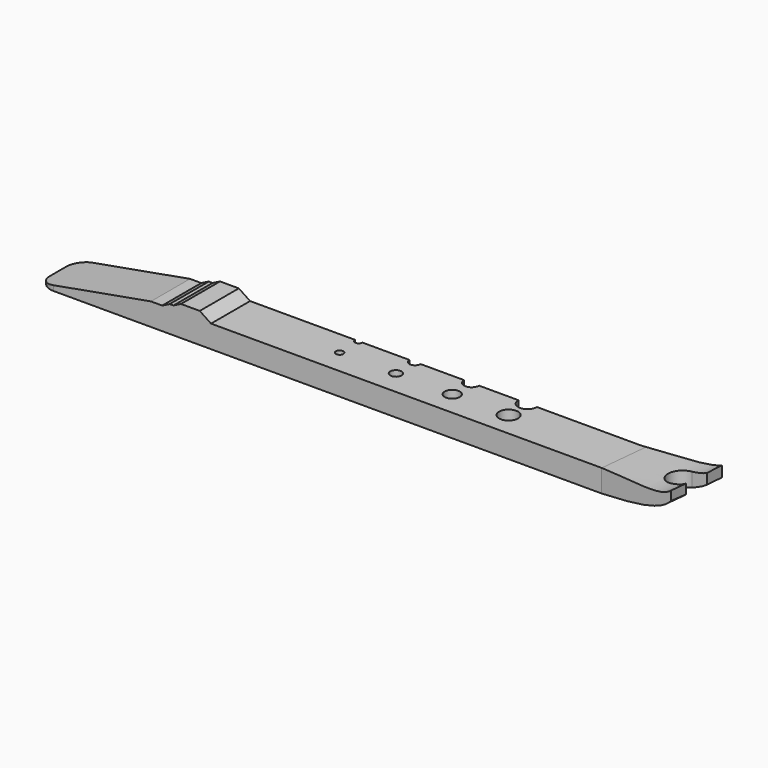
from build123d import *

# Parameters (mm, degrees)
F0_R     = 1
F0_R_2   = 1.5
F0_R_3   = 2
F1_DEPTH = 6
F3_DEPTH = 8
F5_DEPTH = 25
F7_DEPTH = 25
F9_DEPTH = 13


# Not quite as in the source:
# - a feature names something its author has since deleted; it is built from what else it names


with BuildPart() as f1:
    # F0 (on Top) → F1 (new body)
    with BuildSketch(Plane.XY):
        with BuildLine():
            Line((-42.1966487169, -12.8954221606), (-42.1966487169, -25.8954221606))
            Line((-42.1966487169, -25.8954221606), (17.9292613268, -25.8954221606))
            Line((17.9292613268, -25.8954221606), (47.9292613268, -25.8954221606))
            Line((47.9292613268, -25.8954221606), (47.9292613268, -12.8954221606))
            Line((47.9292613268, -12.8954221606), (20.3033512831, -12.8954221606))
            ThreePointArc((20.3033512831, -12.8954221606), (17.8033512831, -15.3954221606), (15.3033512831, -12.8954221606))
            Line((15.3033512831, -12.8954221606), (4.8663063049, -12.8954221606))
            ThreePointArc((4.8663063049, -12.8954221606), (2.8663063049, -14.8954221606), (0.8663063049, -12.8954221606))
            Line((0.8663063049, -12.8954221606), (-10.6966487169, -12.8954221606))
            ThreePointArc((-10.6966487169, -12.8954221606), (-12.1966487169, -14.3954221606), (-13.6966487169, -12.8954221606))
            Line((-13.6966487169, -12.8954221606), (-26.1966487169, -12.8954221606))
            ThreePointArc((-26.1966487169, -12.8954221606), (-27.1966487169, -13.8954221606), (-28.1966487169, -12.8954221606))
            Line((-28.1966487169, -12.8954221606), (-42.1966487169, -12.8954221606))
        make_face()
        with Locations((-27.0707386732, -19.3954221606)):
            Circle(F0_R, mode=Mode.SUBTRACT)
        with Locations((-12.0707386732, -19.3954221606)):
            Circle(F0_R_2, mode=Mode.SUBTRACT)
        with Locations((2.9292613268, -19.3954221606)):
            Circle(F0_R_3, mode=Mode.SUBTRACT)
        with BuildLine():
            ThreePointArc((20.4292613268, -19.3954221606), (19.6970282798, -21.1631891136), (17.9292613268, -21.8954221606))
            ThreePointArc((17.9292613268, -21.8954221606), (16.1614943738, -17.6276552077), (20.4292613268, -19.3954221606))
        make_face(mode=Mode.SUBTRACT)
        with BuildLine():
            ThreePointArc((-102.1092408178, -21.9157785711), (-100.9305134828, -24.7310372299), (-98.109292616, -25.8954221606))
            Line((-98.109292616, -25.8954221606), (-42.1966487169, -25.8954221606))
            Line((-42.1966487169, -25.8954221606), (-42.1966487169, -12.8954221606))
            Line((-42.1966487169, -12.8954221606), (-98.1347384587, -12.8954221606))
            ThreePointArc((-98.1347384587, -12.8954221606), (-100.9703535279, -14.0742012939), (-102.1346866604, -16.9157785711))
            Line((-102.1346866604, -16.9157785711), (-102.1092408178, -21.9157785711))
        make_face()
    extrude(amount=F1_DEPTH)

    # F2 (on face) → F3 (join)
    with BuildSketch(Plane(origin=(0, 0, 0), x_dir=(1, 0, 0), z_dir=(0, 0, -1))):
        with BuildLine():
            Line((47.9292613268, 25.8954221606), (47.9292613268, 12.8954221606))
            Line((47.9292613268, 12.8954221606), (67.9292613268, 10.8954221606))
            Line((67.9292613268, 10.8954221606), (67.9292613268, 15.8954221606))
            Line((67.9292613268, 15.8954221606), (63.9292613268, 15.8954221606))
            ThreePointArc((63.9292613268, 15.8954221606), (60.4292613268, 19.3954221606), (63.9292613268, 22.8954221606))
            Line((63.9292613268, 22.8954221606), (67.9292613268, 22.8954221606))
            Line((67.9292613268, 22.8954221606), (67.9292613268, 27.8954221606))
            Line((67.9292613268, 27.8954221606), (47.9292613268, 25.8954221606))
        make_face()
    extrude(amount=-F3_DEPTH)

    # F4 (on face) → F5 (cut)
    with BuildSketch(Plane(origin=(-2.0893560424, -20.8935604237, 0), x_dir=(0.9950371902, -0.099503719, 0), z_dir=(-0.099503719, -0.9950371902, 0))):
        with BuildLine():
            Line((47.7105565369, 6), (50.2680883301, 6))
            Line((50.2680883301, 6), (50.2680883301, 8))
            Line((50.2680883301, 8), (70.3678395723, 8))
            add(Edge.make_bspline(
                [(70.3678395723, 8), (72.5767643682, 9.8820103785), (72.4269967916, 13.5723014467), (72.296127677, 17.0164462179)],
                knots=[0.596790788, 0.596790788, 0.596790788, 0.596790788, 1, 1, 1, 1], degree=3))
            add(Edge.make_bspline(
                [(70.3678395723, 5.5720340461), (72.8712183365, 8.3489220533), (72.5836730067, 12.6826841356), (72.296127677, 17.0164462179)],
                knots=[0.5727584581, 0.5727584581, 0.5727584581, 0.5727584581, 1, 1, 1, 1], degree=3))
            Line((70.3678395723, 5.5720340461), (70.3678395723, 0))
            Line((70.3678395723, 0), (50.2680883301, 0))
            Line((50.2680883301, 0), (50.2680883301, -3.928697668))
            Line((50.2680883301, -3.928697668), (74.866913259, -3.928697668))
            Line((74.866913259, -3.928697668), (74.866913259, 21.5322930813))
            Line((74.866913259, 21.5322930813), (50.2680883301, 21.5322930813))
            Line((50.2680883301, 21.5322930813), (47.7105565369, 21.5322930813))
            Line((47.7105565369, 21.5322930813), (47.7105565369, 6))
        make_face()
        with BuildLine():
            Line((50.2680883301, 8), (50.2680883301, 6))
            add(Edge.make_bspline(
                [(50.2680883301, 6), (58.6617788579, 6.3902694532), (67.098405416, 5.2144325486), (70.3678395723, 8)],
                knots=[0, 0, 0, 0, 0.596790788, 0.596790788, 0.596790788, 0.596790788], degree=3))
            Line((70.3678395723, 8), (50.2680883301, 8))
        make_face()
        with BuildLine():
            add(Edge.make_bspline(
                [(50.2680883301, 0), (58.6399537153, 0.9246740387), (67.0118191006, 1.8493480774), (70.3678395723, 5.5720340461)],
                knots=[0, 0, 0, 0, 0.5727584581, 0.5727584581, 0.5727584581, 0.5727584581], degree=3))
            Line((50.2680883301, 0), (70.3678395723, 0))
            Line((70.3678395723, 0), (70.3678395723, 5.5720340461))
        make_face()
    extrude(amount=-F5_DEPTH, mode=Mode.SUBTRACT)

    # F6 (on face) → F7 (cut)
    with BuildSketch(Plane.XZ.offset(25.8954221606)):
        Polygon((-103.6658883095, 0), (-101.9829884171, 0.653559342), (-72.109292616, 6), (-72.109292616, 8.9457267895), (-103.4941226244, 6.6766636446), align=None)
    extrude(amount=-F7_DEPTH, mode=Mode.SUBTRACT)

    # F8 (on face) → F9 (join)
    with BuildSketch(Plane.XZ.offset(25.8954221606)):
        Polygon((-67.109292616, 7), (-69.109292616, 6), (-67.109292616, 6), (-56.109292616, 6), (-59.109292616, 8), (-64.109292616, 8), (-66.109292616, 7), align=None)
    extrude(amount=-F9_DEPTH)


solid = f1.part
